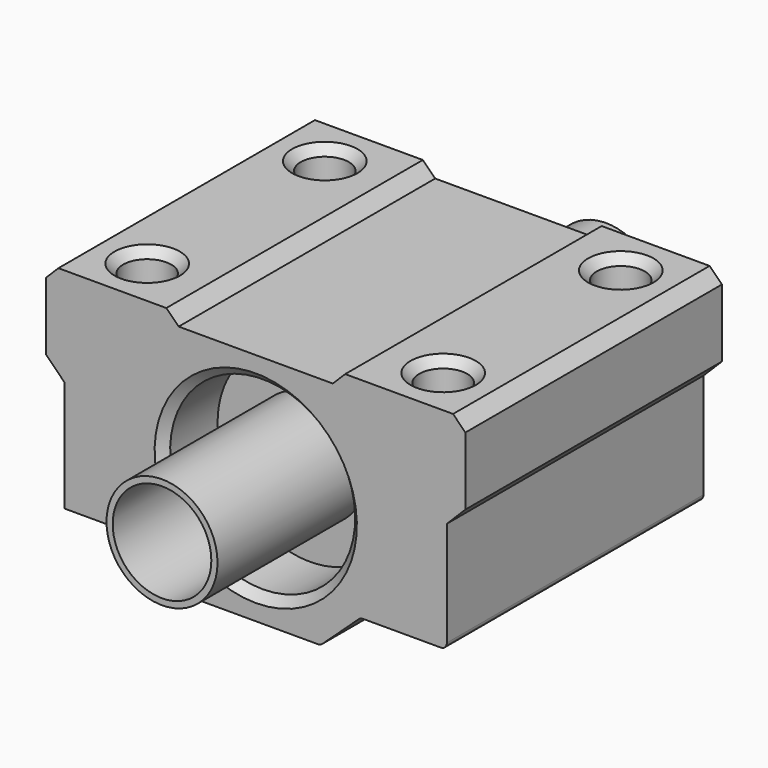
from build123d import *

# Parameters (mm, degrees)
F1_DEPTH       = 13
F2_SIZE        = 0.99999
F3_SIZE        = 1.49999
F4_R           = 0.5
F6_D           = 3.6
F6_CBORE_D     = 3.9
F6_CBORE_DEPTH = 6
F7_SIZE        = 0.7
F0_R           = 4.5
F8_DEPTH       = 7.5
F0_R_2         = 4
F9_DEPTH       = 22.5


# Not quite as in the source:
# - a fillet or chamfer is up to 0.001 mm smaller than in the source, because OpenCascade refuses the exact size


with BuildPart() as f1:
    # F0 (on Front) → F1 (new body, symmetric)
    with BuildSketch(Plane.XZ):
        with BuildLine():
            ThreePointArc((0, 7.5), (5.3033008589, 5.3033008589), (7.5, 0))
            ThreePointArc((7.5, 0), (5.3033008589, -5.3033008589), (0, -7.5))
            Line((0, -7.5), (0, -9.5))
            Line((0, -9.5), (5.25, -9.5))
            Line((5.25, -9.5), (8.5, -6.5))
            Line((8.5, -6.5), (15.5, -6.5))
            Line((15.5, -6.5), (15.5, 2.5))
            Line((15.5, 2.5), (17, 2.5))
            Line((17, 2.5), (17, 10.5))
            Line((17, 10.5), (7.25, 10.5))
            Line((7.25, 10.5), (7.25, 9.5))
            Line((7.25, 9.5), (0, 9.5))
            Line((0, 9.5), (0, 7.5))
        make_face()
        with BuildLine():
            ThreePointArc((0, -7.5), (-7.5, 0), (0, 7.5))
            Line((0, 7.5), (0, 9.5))
            Line((0, 9.5), (-7.25, 9.5))
            Line((-7.25, 9.5), (-7.25, 10.5))
            Line((-7.25, 10.5), (-17, 10.5))
            Line((-17, 10.5), (-17, 2.5))
            Line((-17, 2.5), (-15.5, 2.5))
            Line((-15.5, 2.5), (-15.5, -6.5))
            Line((-15.5, -6.5), (-8.5, -6.5))
            Line((-8.5, -6.5), (-5.25, -9.5))
            Line((-5.25, -9.5), (0, -9.5))
            Line((0, -9.5), (0, -7.5))
        make_face()
    extrude(amount=F1_DEPTH, both=True)

    # F2 (size 1 in the source; OpenCascade refuses exactly that, so slightly less here)
    f2_edges = [f1.edges().sort_by_distance(p)[0] for p in [
        (7.25, 0, 9.5),
        (17, 0, 10.5),
        (-7.25, 0, 9.5),
        (-17, 0, 10.5),
    ]]
    chamfer(f2_edges, length=F2_SIZE)

    # F3 (size 1.5 in the source; OpenCascade refuses exactly that, so slightly less here)
    f3_edges = [f1.edges().sort_by_distance(p)[0] for p in [
        (17, 0, 2.5),
        (-17, 0, 2.5),
    ]]
    chamfer(f3_edges, length=F3_SIZE)

    # F4
    f4_edges = [f1.edges().sort_by_distance(p)[0] for p in [
        (15.5, 0, -6.5),
        (8.5, 0, -6.5),
        (5.25, 0, -9.5),
        (-5.25, 0, -9.5),
        (-8.5, 0, -6.5),
    ]]
    fillet(f4_edges, radius=F4_R)

    # F6 (through all)
    with Locations(Plane.XY.offset(10.5)):
        with Locations((12, 9), (12, -9), (-12, 9), (-12, -9)):
            CounterBoreHole(F6_D / 2, F6_CBORE_D / 2, F6_CBORE_DEPTH)

    # F7
    f7_edges = [f1.edges().sort_by_distance(p)[0] for p in [
        (-7.5, -13, 0),
        (-7.5, 13, 0),
        (10.05, 9, 10.5),
        (10.05, -9, 10.5),
        (-13.95, 9, 10.5),
        (-13.95, -9, 10.5),
    ]]
    chamfer(f7_edges, length=F7_SIZE)


with BuildPart() as f8:
    # F0 (on Front) → F8 (new body, symmetric)
    with BuildSketch(Plane.XZ):
        with BuildLine():
            ThreePointArc((0, -7.5), (5.3033008589, -5.3033008589), (7.5, 0))
            ThreePointArc((7.5, 0), (5.3033008589, 5.3033008589), (0, 7.5))
            ThreePointArc((0, 7.5), (-7.5, 0), (0, -7.5))
        make_face()
        Circle(F0_R, mode=Mode.SUBTRACT)
    extrude(amount=F8_DEPTH, both=True)

    # F0 (on Front) → F9 (join, symmetric)
    with BuildSketch(Plane.XZ):
        Circle(F0_R)
        Circle(F0_R_2, mode=Mode.SUBTRACT)
    extrude(amount=F9_DEPTH, both=True)


solid = Compound([f1.part, f8.part])
